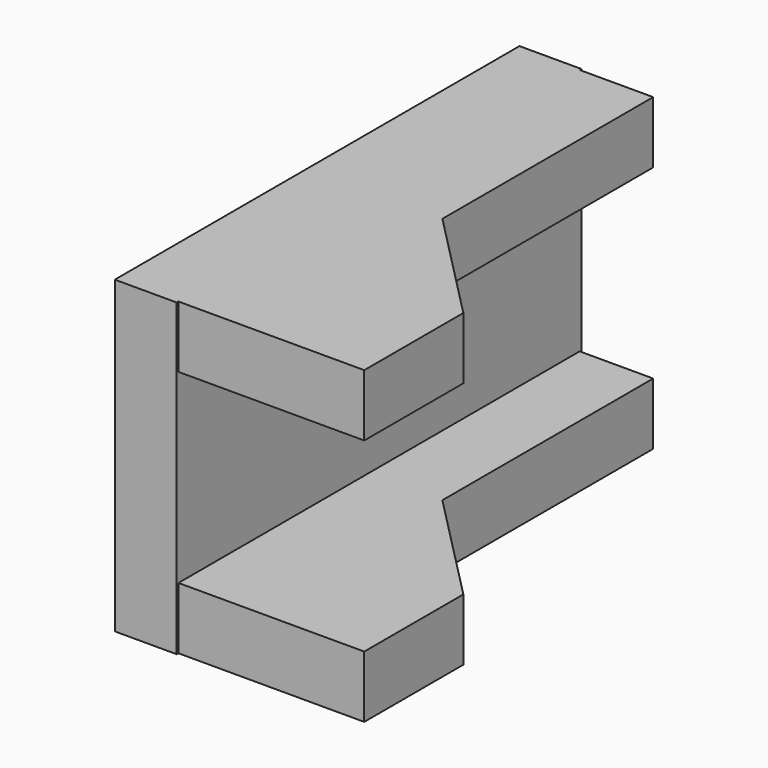
from build123d import *

# Parameters (mm, degrees)
F0_W     = 77.7875
F0_H     = 47.625
F1_DEPTH = 9.525
F2_R     = 12.6438150781
F3_DEPTH = 97
F5_DEPTH = 9.525


# Not quite as in the source:
# - an extrude ends at something that could not be found from the text; its depth is read off the source's solid


with BuildPart() as f1:
    # F0 (on Right) → F1 (new body)
    with BuildSketch(Plane.YZ):
        Rectangle(F0_W, F0_H)
    extrude(amount=F1_DEPTH)

    # F2 (on Right) → F3 (cut, through all)
    with BuildSketch(Plane.YZ):
        Circle(F2_R)
    extrude(amount=-F3_DEPTH, mode=Mode.SUBTRACT)

    # F4 (on face) → F5 (join)
    with BuildSketch(Plane.XY.offset(23.8125)):
        Polygon((0, 38.5659709573), (0, -38.5659709573), (38.1, -38.5659709573), (38.1, -19.5159709573), (20.8316552401, -1.9598177195), (20.8316552401, 38.5659709573), align=None)
    extrude(amount=-F5_DEPTH)

    # F6: F1 across plane


with BuildPart() as f1_1:
    add(f1.part)
    add(f1.part.mirror(Plane.XY))


solid = f1_1.part
